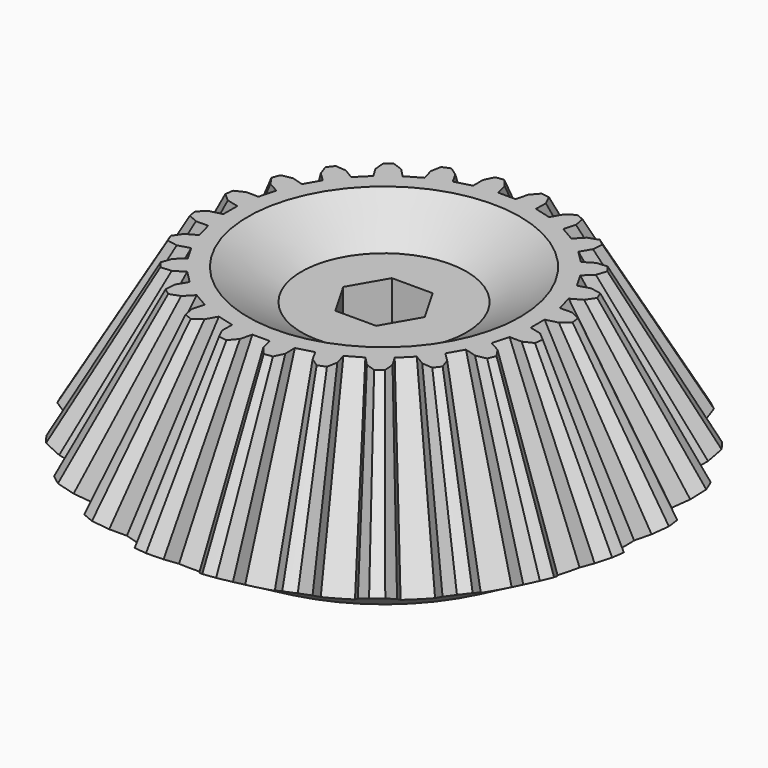
from build123d import *

# Parameters (mm, degrees)
F4_COPIES_COUNT = 24
F8_DEPTH        = 15.001


# Not quite as in the source:
# - a pattern or mirror of a feature is missing from the dataset's text; its kind, count and spacing are read off the source's solid
# - a feature names something its author has since deleted; it is built from what else it names


with BuildPart() as f1:
    # F0 (on Front) → F1 (revolve)
    with BuildSketch(Plane.XZ):
        Polygon((14.6076951546, 0), (22.4019237886, 4.5), (0, 43.3012701892), (0, 0), align=None)
    revolve(axis=Axis((0, 0, 21.6506350946), (0, 0, -1)))

    # F3 (on line) → F4 section 0
    with BuildSketch(Plane(origin=(3.6519237886, 0, -6.3253175473), x_dir=(0.8660254038, 0, 0.5), z_dir=(-0.5, 0, 0.8660254038)), mode=Mode.PRIVATE) as f4_s0:
        Polygon((20.6230163694, -1.5178986274), (21.6506350946, -2.5), (21.6506350946, 2.5), (20.6230163694, 1.5178986274), (19.25, 1.15), (19.25, 0), (19.25, -1.15), align=None)
    f4 = loft([f4_s0.sketch, Vertex(0, 0, 43.3012701892)], mode=Mode.SUBTRACT)

    # F4_copies: F4 ×24 about axis
    f4_copies_axis = Axis((0, 0, 0), (0, 0, 1))
    for i in range(1, F4_COPIES_COUNT):
        add(f4.rotate(f4_copies_axis, i * 360 / F4_COPIES_COUNT), mode=Mode.SUBTRACT)

    # F5 (on Front) → F6 (revolve, cut)
    with BuildSketch(Plane.XZ):
        Polygon((0, 46.7511937022), (0, 15), (7, 15), (11.5466333699, 17.625), (17.5466333699, 17.625), align=None)
    revolve(axis=Axis((0, 0, 30.8755968511), (0, 0, -1)), mode=Mode.SUBTRACT)

    # F7 (on face) → F8 (cut, through all)
    with BuildSketch(Plane.XY.offset(15)):
        Polygon((1.7320508076, 3), (-1.7320508076, 3), (-3.4641016151, 0), (-1.7320508076, -3), (1.7320508076, -3), (3.4641016151, 0), align=None)
    extrude(amount=-F8_DEPTH, mode=Mode.SUBTRACT)


solid = f1.part
